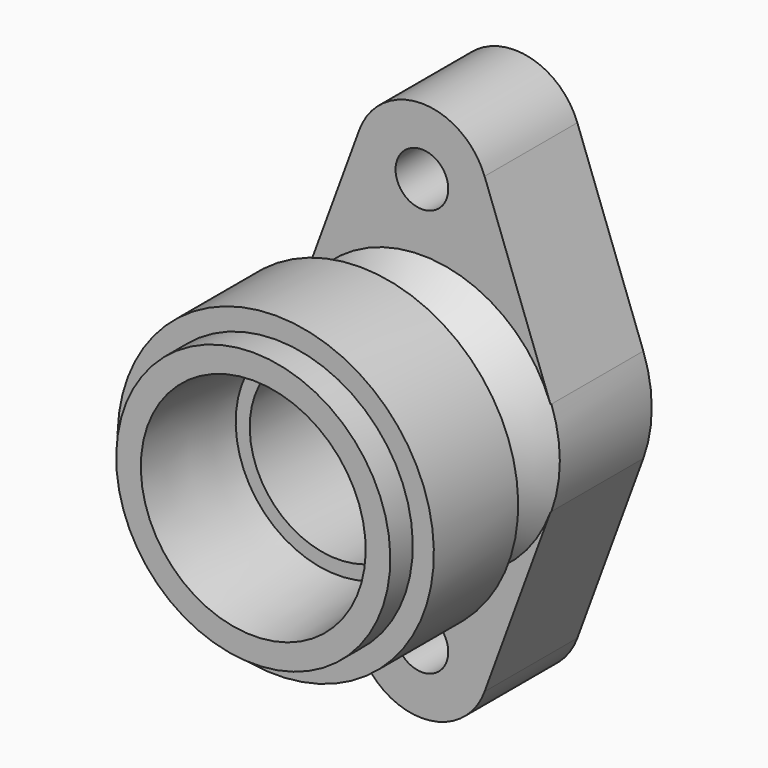
from build123d import *

# Parameters (mm, degrees)
F2_R     = 7.5
F4_DEPTH = 33


# Not quite as in the source:
# - a feature of the source that left no trace in its solid (it failed there, or was rolled back) is left out


with BuildPart() as f1:
    # F0 (on Right) → F1 (revolve)
    with BuildSketch(Plane.YZ):
        with BuildLine():
            Line((-13.5163067589, 39), (-21.5163067589, 39))
            Line((-21.5163067589, 39), (-21.5163067589, 32))
            Line((-21.5163067589, 32), (8.4836932411, 29))
            Line((8.4836932411, 29), (8.4836932411, 25))
            Line((8.4836932411, 25), (50.4836932411, 25))
            Line((50.4836932411, 25), (50.4836932411, 0))
            Line((50.4836932411, 0), (68.4836932411, 0))
            Line((68.4836932411, 0), (68.4836932411, 32))
            Line((68.4836932411, 32), (71.4836932411, 32))
            Line((71.4836932411, 32), (71.4836932411, 39))
            Line((71.4836932411, 39), (38.7984625995, 39))
            Line((38.7984625995, 39), (24.3515754229, 28.8841806952))
            ThreePointArc((24.3515754229, 28.8841806952), (19.1749501749, 28.5448867508), (16.4836932411, 32.9799409167))
            Line((16.4836932411, 32.9799409167), (16.4836932411, 45))
            Line((16.4836932411, 45), (-13.5163067589, 45))
            Line((-13.5163067589, 45), (-13.5163067589, 39))
        make_face()
    revolve(axis=Axis((0, 59.4836932411, 0), (0, -1, 0)))

    # F2 (on face) → F4 (join)
    with BuildSketch(Plane(origin=(0, 71.4836932411, 0), x_dir=(-1, 0, 0), z_dir=(0, 1, 0))):
        with BuildLine():
            ThreePointArc((36.6079755837, -13.4482758621), (0, -39), (-36.6079755837, -13.4482758621))
            Line((-36.6079755837, -13.4482758621), (-17.8346547716, -64.5517241379))
            ThreePointArc((-17.8346547716, -64.5517241379), (0, -77), (17.8346547716, -64.5517241379))
            Line((17.8346547716, -64.5517241379), (36.6079755837, -13.4482758621))
        make_face()
        with Locations((0, -58)):
            Circle(F2_R, mode=Mode.SUBTRACT)
        with BuildLine():
            ThreePointArc((17.8346547716, 64.5517241379), (0, 77), (-17.8346547716, 64.5517241379))
            Line((-17.8346547716, 64.5517241379), (-36.6079755837, 13.4482758621))
            ThreePointArc((-36.6079755837, 13.4482758621), (0, 39), (36.6079755837, 13.4482758621))
            Line((36.6079755837, 13.4482758621), (17.8346547716, 64.5517241379))
        make_face()
        with Locations((0, 58)):
            Circle(F2_R, mode=Mode.SUBTRACT)
    extrude(amount=-F4_DEPTH)


solid = f1.part
